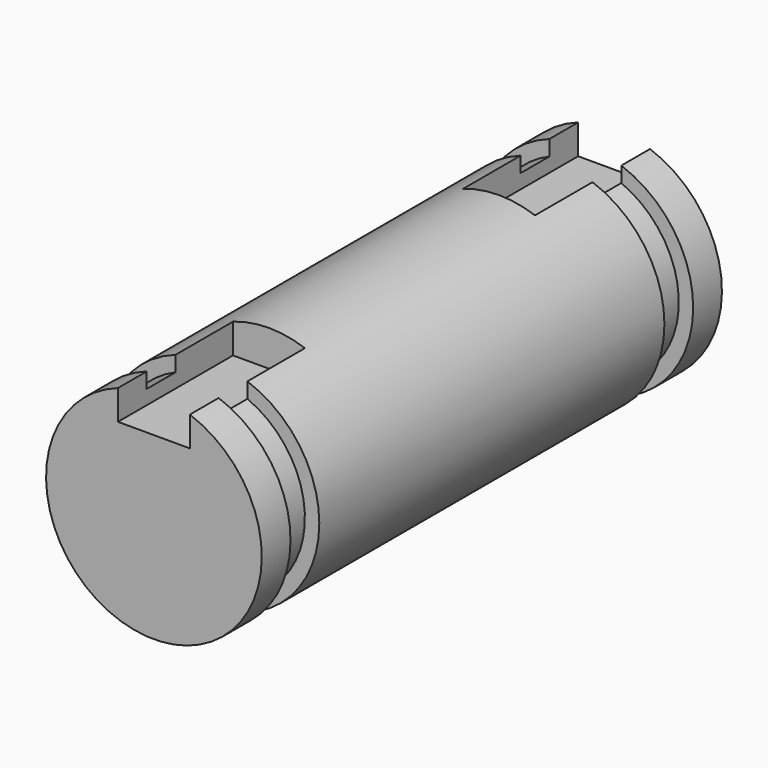
from build123d import *

# Parameters (mm, degrees)
F0_R            = 4.7625
F1_DEPTH        = 25.4
F2_W            = 3.175
F2_H            = 3.175
F3_DEPTH        = 6.35
F3_COPIES_COUNT = 2
F3_COPIES_PITCH = 19.05
F5_W            = 1.5875
F5_H            = 0.635


# Not quite as in the source:
# - a pattern or mirror of a feature is missing from the dataset's text; its kind, count and spacing are read off the source's solid


with BuildPart() as f1:
    # F0 (on Front) → F1 (new body)
    with BuildSketch(Plane.XZ):
        Circle(F0_R)
    extrude(amount=F1_DEPTH)

    # F2 (on face) → F3 (cut)
    with BuildSketch(Plane.XZ.offset(25.4)):
        with Locations((0, 4.7625)):
            Rectangle(F2_W, F2_H)
    f3 = extrude(amount=-F3_DEPTH, mode=Mode.SUBTRACT)

    # F3_copies: F3 ×2
    with Locations(*[(0, i * F3_COPIES_PITCH, 0) for i in range(1, F3_COPIES_COUNT)]):
        add(f3, mode=Mode.SUBTRACT)

    # F5 (on Right) → F6 (revolve, cut)
    with BuildSketch(Plane.YZ):
        with Locations((-23.01875, -4.445)):
            Rectangle(F5_W, F5_H)
    f6 = revolve(axis=Axis((0, -12.6913171262, 0), (0, 1, 0)), mode=Mode.SUBTRACT)

    # F6_copies: F6 across plane
    add(f6.mirror(Plane.ZX.offset(-12.7)), mode=Mode.SUBTRACT)


solid = f1.part
